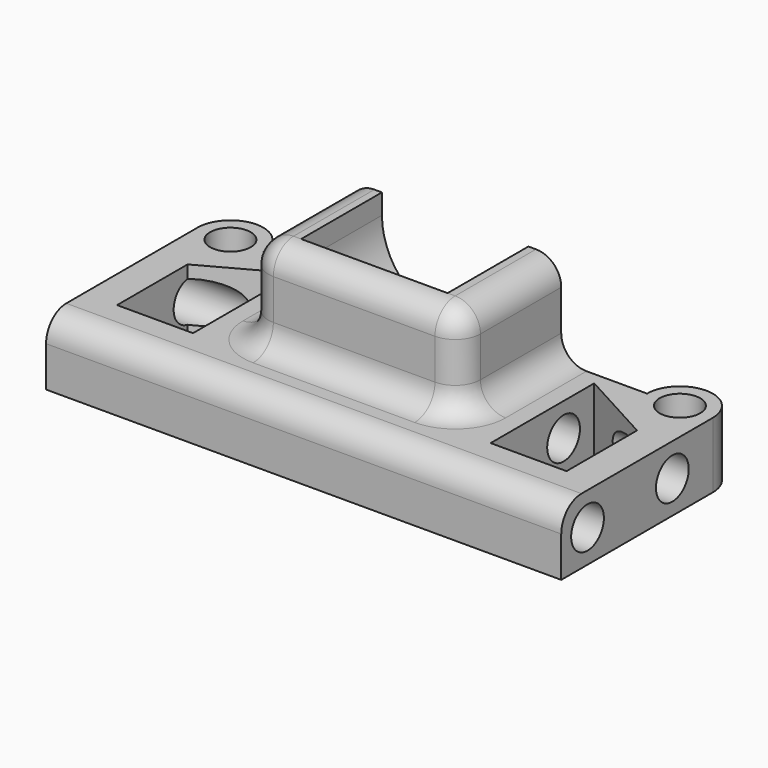
from build123d import *

# Parameters (mm, degrees)
F0_R      = 4.025
F1_DEPTH  = 13
F2_R      = 4.05
F3_DEPTH  = 120
F5_DEPTH  = 18
F6_R      = 1.25
F7_DEPTH  = 20
F8_R      = 4.99999
F10_DEPTH = 25


# Not quite as in the source:
# - a fillet or chamfer is up to 0.001 mm smaller than in the source, because OpenCascade refuses the exact size


with BuildPart() as f1:
    # F0 (on Top) → F1 (new body)
    with BuildSketch(Plane.XY):
        with BuildLine():
            Line((38, 0), (0, 0))
            Line((0, 0), (-38, 0))
            ThreePointArc((-38, 0), (-44.5, 6.5), (-51, 0))
            Line((-51, 0), (-51, -37.5))
            Line((-51, -37.5), (0, -37.5))
            Line((0, -37.5), (51, -37.5))
            Line((51, -37.5), (51, 0))
            ThreePointArc((51, 0), (44.5, 6.5), (38, 0))
        make_face()
        with Locations((-44.5, 0)):
            Circle(F0_R, mode=Mode.SUBTRACT)
        with Locations((44.5, 0)):
            Circle(F0_R, mode=Mode.SUBTRACT)
    extrude(amount=F1_DEPTH)

    # F2 (on face) → F3 (cut)
    with BuildSketch(Plane.YZ.offset(51)):
        with Locations((-31, 6.5)):
            Circle(F2_R)
        with Locations((-10, 6.5)):
            Circle(F2_R)
    extrude(amount=-F3_DEPTH, mode=Mode.SUBTRACT)

    # F4 (on face) → F5 (join)
    with BuildSketch(Plane.XY.offset(13)):
        Polygon((-21, -25), (0, -25), (21, -25), (21, 0), (-21, 0), align=None)
    extrude(amount=F5_DEPTH)

    # F6 (on face) → F7 (cut)
    with BuildSketch(Plane(origin=(0, 0, 0), x_dir=(-1, 0, 0), z_dir=(0, 1, 0))):
        with BuildLine():
            Line((-14.5, 31), (-14.5, 27))
            ThreePointArc((-14.5, 27), (0, 12.5), (14.5, 27))
            Line((14.5, 27), (14.5, 31))
            Line((14.5, 31), (-14.5, 31))
        make_face()
        with Locations((-16.4399370551, 27)):
            Circle(F6_R)
        with Locations((16.4399370551, 27)):
            Circle(F6_R)
    extrude(amount=-F7_DEPTH, mode=Mode.SUBTRACT)

    # F8 (radius 5 in the source; OpenCascade refuses exactly that, so slightly less here)
    f8_edges = [f1.edges().sort_by_distance(p)[0] for p in [
        (21, -12.5, 31),
        (-21, -12.5, 31),
        (21, -12.5, 13),
        (-21, -12.5, 13),
        (0, -25, 31),
        (21, -25, 22),
        (-21, -25, 22),
        (0, -37.5, 13),
        (0, -25, 13),
    ]]
    fillet(f8_edges, radius=F8_R)

    # F9 (on face) → F10 (cut)
    with BuildSketch(Plane.XY.offset(13)):
        Polygon((44.5, -28.0575975776), (44.5, -10.6131481007), (29.4615291059, -2.4116530549), (29.4615291059, -28.0575975776), align=None)
        Polygon((-29.4615291059, -2.4116530549), (-44.5, -10.6131481007), (-44.5, -28.0575975776), (-29.4615291059, -28.0575975776), align=None)
    extrude(amount=-F10_DEPTH, mode=Mode.SUBTRACT)


solid = f1.part
